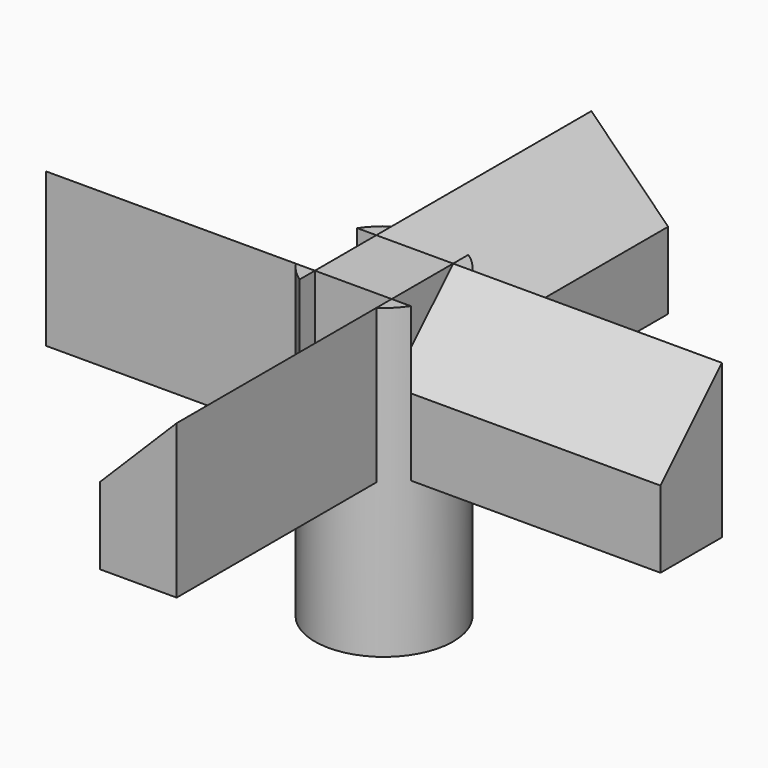
from build123d import *

# Parameters (mm, degrees)
F0_R     = 4.5
F1_DEPTH = 10
F2_W     = 5
F2_H     = 5
F3_DEPTH = 10
F4_SIZE  = 4.99999
F5_DEPTH = 10
F7_D     = 2
F7_DEPTH = 9
F7_TIP   = 0.600860619


# Not quite as in the source:
# - a fillet or chamfer is up to 0.001 mm smaller than in the source, because OpenCascade refuses the exact size


with BuildPart() as f1:
    # F0 (on Top) → F1 (new body)
    with BuildSketch(Plane.XY):
        Circle(F0_R)
    extrude(amount=F1_DEPTH)

    # F2 (on face) → F3 (join)
    with BuildSketch(Plane.XY.offset(10)):
        with BuildLine():
            ThreePointArc((2.5, -3.7416573868), (0, -4.5), (-2.5, -3.7416573868))
            Line((-2.5, -3.7416573868), (-2.5, -20))
            Line((-2.5, -20), (2.5, -20))
            Line((2.5, -20), (2.5, -3.7416573868))
        make_face()
        with BuildLine():
            Line((-3.7416573868, 2.5), (-20, 2.5))
            Line((-20, 2.5), (-20, -2.5))
            Line((-20, -2.5), (-3.7416573868, -2.5))
            ThreePointArc((-3.7416573868, -2.5), (-4.5, 0), (-3.7416573868, 2.5))
        make_face()
        with BuildLine():
            Line((-2.5, 20), (-2.5, 3.7416573868))
            ThreePointArc((-2.5, 3.7416573868), (0, 4.5), (2.5, 3.7416573868))
            Line((2.5, 3.7416573868), (2.5, 20))
            Line((2.5, 20), (-2.5, 20))
        make_face()
        with BuildLine():
            Line((20, 2.5), (3.7416573868, 2.5))
            ThreePointArc((3.7416573868, 2.5), (4.3062430401, 1.3062430401), (4.5, 0))
            ThreePointArc((4.5, 0), (4.3062430401, -1.3062430401), (3.7416573868, -2.5))
            Line((3.7416573868, -2.5), (20, -2.5))
            Line((20, -2.5), (20, 2.5))
        make_face()
        with BuildLine():
            Line((3.7416573868, 2.5), (2.5, 2.5))
            Line((2.5, 2.5), (2.5, -2.5))
            Line((2.5, -2.5), (3.7416573868, -2.5))
            ThreePointArc((3.7416573868, -2.5), (4.3062430401, -1.3062430401), (4.5, 0))
            ThreePointArc((4.5, 0), (4.3062430401, 1.3062430401), (3.7416573868, 2.5))
        make_face()
        Rectangle(F2_W, F2_H)
        with BuildLine():
            Line((2.5, -2.5), (-2.5, -2.5))
            Line((-2.5, -2.5), (-2.5, -3.7416573868))
            ThreePointArc((-2.5, -3.7416573868), (0, -4.5), (2.5, -3.7416573868))
            Line((2.5, -3.7416573868), (2.5, -2.5))
        make_face()
        with BuildLine():
            Line((-2.5, 2.5), (-3.7416573868, 2.5))
            ThreePointArc((-3.7416573868, 2.5), (-4.5, 0), (-3.7416573868, -2.5))
            Line((-3.7416573868, -2.5), (-2.5, -2.5))
            Line((-2.5, -2.5), (-2.5, 2.5))
        make_face()
        with BuildLine():
            Line((-2.5, 3.7416573868), (-2.5, 2.5))
            Line((-2.5, 2.5), (2.5, 2.5))
            Line((2.5, 2.5), (2.5, 3.7416573868))
            ThreePointArc((2.5, 3.7416573868), (0, 4.5), (-2.5, 3.7416573868))
        make_face()
    extrude(amount=F3_DEPTH)

    # F4 (size 5 in the source; OpenCascade refuses exactly that, so slightly less here)
    f4_edges = [f1.edges().sort_by_distance(p)[0] for p in [
        (-2.5, -11.25, 20),
        (-11.25, 2.5, 20),
        (2.5, 11.25, 20),
        (11.25, -2.5, 20),
    ]]
    chamfer(f4_edges, length=F4_SIZE)

    # F5 (add): faces of the model
    f5_faces = [f1.faces().sort_by_distance(p)[0] for p in [
        (-2.940797231, 2.940797231, 10),
        (2.940797231, 2.940797231, 10),
        (2.940797231, -2.940797231, 10),
        (-2.940797231, -2.940797231, 10),
    ]]
    extrude(f5_faces, amount=F5_DEPTH)

    # F7
    with Locations(Plane(origin=(0, 0, 0), x_dir=(1, 0, 0), z_dir=(0, 0, -1))):
        with Locations((0, 0)):
            Hole(F7_D / 2, depth=F7_DEPTH)
            with Locations((0, 0, -(F7_DEPTH + F7_TIP / 2))):  # 118° drill point
                Cone(0, F7_D / 2, F7_TIP, mode=Mode.SUBTRACT)


solid = f1.part
